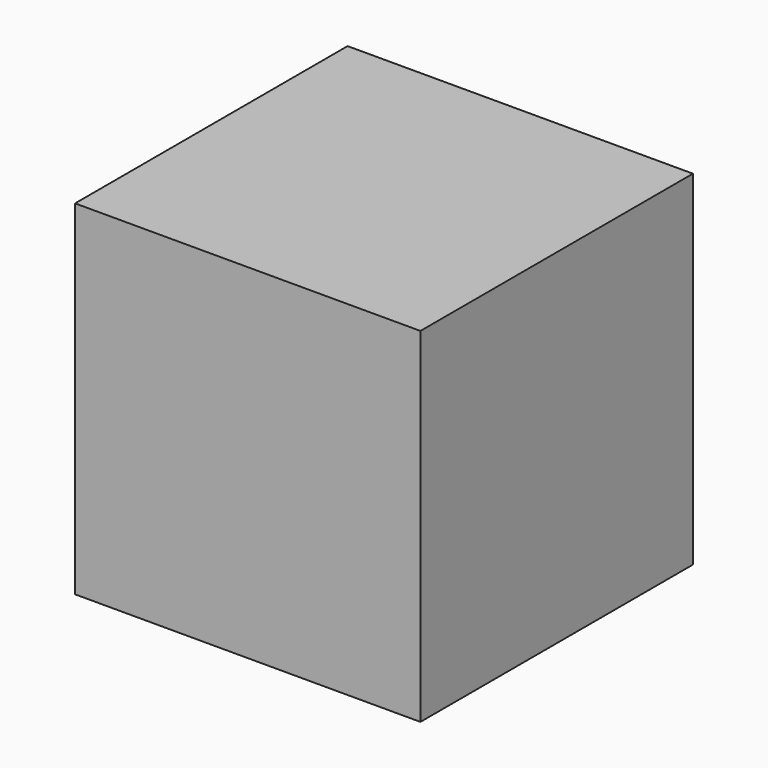
from build123d import *

# Parameters (mm, degrees)
F0_W     = 103.0072718859
F0_H     = 102.6731655002
F1_DEPTH = 101.6


# Not quite as in the source:
# - the program builds the solid bodies; features that only make, move or delete a surface that nothing else refers to are left out


with BuildPart() as f1:
    # F0 (on Front) → F1 (new body)
    with BuildSketch(Plane.XZ):
        with Locations((-51.5036359429, 51.3365827501)):
            Rectangle(F0_W, F0_H)
    extrude(amount=F1_DEPTH)


solid = f1.part
